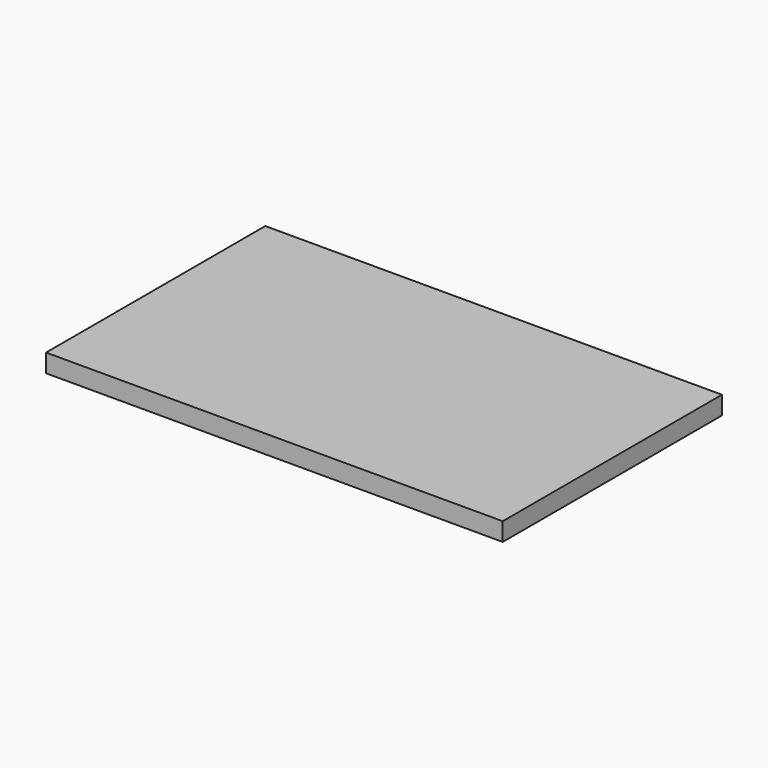
from build123d import *

# Parameters (mm, degrees)
F0_W     = 250
F0_H     = 150
F1_DEPTH = 10


# Not quite as in the source:
# - a feature names something its author has since deleted; it is built from what else it names


with BuildPart() as f1:
    # F0 (on Top) → F1 (new body)
    with BuildSketch(Plane.XY):
        with Locations((125, 75)):
            Rectangle(F0_W, F0_H)
    extrude(amount=-F1_DEPTH)


solid = f1.part
